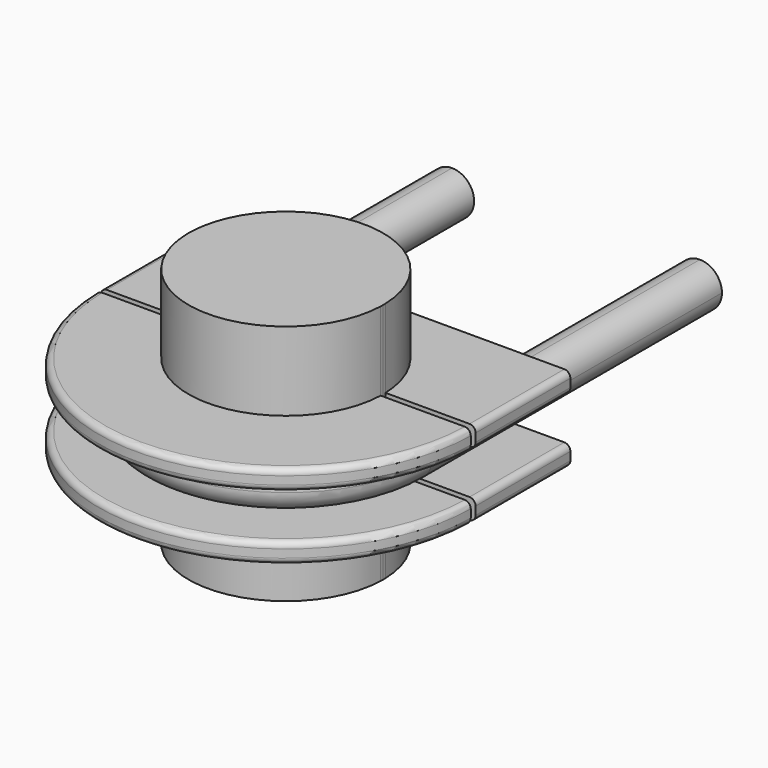
from build123d import *

# Parameters (mm, degrees)
F0_W          = 10.4959674797
F0_H          = 19.6
F4_DEPTH      = 7
F4_DEPTH_BACK = 7
F6_R          = 1
F6_2_R        = 1


with BuildPart() as f2:
    # F2: sweep along a path in F0
    with BuildLine(Plane.XY) as f2_path:
        Line((-20.5, 60), (-20.5, 0))
        ThreePointArc((-20.5, 0), (0, -20.5), (20.5, 0))
        Line((20.5, 0), (20.5, 60))
    # F1 (on Front) → F2 (sweep)
    with BuildSketch(Plane.XZ):
        with BuildLine():
            ThreePointArc((20.5, -3.65), (23.0809397513, -2.5809397513), (24.15, 0))
            ThreePointArc((24.15, 0), (23.0809397513, 2.5809397513), (20.5, 3.65))
            ThreePointArc((20.5, 3.65), (16.85, 0), (20.5, -3.65))
        make_face()
    sweep(path=f2_path.line)


with BuildPart() as f3:
    # F3: sweep along a path in F1
    with BuildLine(Plane.XZ) as f3_path:
        Line((0, -20), (0, 0))
        Line((0, 0), (0, 20))
    # F0 (on Top) → F3 (sweep)
    with BuildSketch(Plane.XY):
        with BuildLine():
            ThreePointArc((-16.0922341519, 0.5), (-16.1, 0), (-16.0922341519, -0.5))
            Line((-16.0922341519, -0.5), (16.0922341519, -0.5))
            ThreePointArc((16.0922341519, -0.5), (16.0980584209, -0.2500301524), (16.1, 0))
            ThreePointArc((16.1, 0), (16.0980584209, 0.2500301524), (16.0922341519, 0.5))
            Line((16.0922341519, 0.5), (-16.0922341519, 0.5))
        make_face()
        with BuildLine():
            ThreePointArc((16.0922341519, 0.5), (0, 16.1), (-16.0922341519, 0.5))
            Line((-16.0922341519, 0.5), (16.0922341519, 0.5))
        make_face()
        with BuildLine():
            Line((16.0922341519, -0.5), (-16.0922341519, -0.5))
            ThreePointArc((-16.0922341519, -0.5), (0, -16.1), (16.0922341519, -0.5))
        make_face()
    sweep(path=f3_path.line)


with BuildPart() as f4:
    # F0 (on Top) → F4 (new body, two sides)
    with BuildSketch(Plane.XY) as f4_sk:
        with BuildLine():
            Line((-20.5, 20.1), (-20.5, 0.5))
            Line((-20.5, 0.5), (-16.0922341519, 0.5))
            ThreePointArc((-16.0922341519, 0.5), (0, 16.1), (16.0922341519, 0.5))
            Line((16.0922341519, 0.5), (20.5, 0.5))
            Line((20.5, 0.5), (20.5, 20.1))
            Line((20.5, 20.1), (-20.5, 20.1))
        make_face()
        with Locations((-25.7479837398, 10.3)):
            Rectangle(F0_W, F0_H)
        with Locations((25.7479837398, 10.3)):
            Rectangle(F0_W, F0_H)
    extrude(amount=F4_DEPTH)
    extrude(f4_sk.sketch, amount=-F4_DEPTH_BACK)


with BuildPart() as f4b:
    # F0 (on Top) → F4, piece 2 (new body, two sides)
    with BuildSketch(Plane.XY) as f4_2_sk:
        with BuildLine():
            Line((-16.0922341519, -0.5), (-20.4939015319, -0.5))
            ThreePointArc((-20.4939015319, -0.5), (0, -20.5), (20.4939015319, -0.5))
            Line((20.4939015319, -0.5), (16.0922341519, -0.5))
            ThreePointArc((16.0922341519, -0.5), (0, -16.1), (-16.0922341519, -0.5))
        make_face()
        with BuildLine():
            ThreePointArc((20.4939015319, -0.5), (0, -20.5), (-20.4939015319, -0.5))
            Line((-20.4939015319, -0.5), (-30.9959674797, -0.5))
            ThreePointArc((-30.9959674797, -0.5), (0, -31), (30.9959674797, -0.5))
            Line((30.9959674797, -0.5), (20.4939015319, -0.5))
        make_face()
    extrude(amount=F4_DEPTH)
    extrude(f4_2_sk.sketch, amount=-F4_DEPTH_BACK)


with BuildPart() as f5_tool:
    # F5: sweep along a path in F0
    with BuildLine(Plane.XY) as f5_path:
        Line((20.5, 60), (20.5, 0))
        ThreePointArc((20.5, 0), (0, -20.5), (-20.5, 0))
        Line((-20.5, 0), (-20.5, 60))
    # F1 (on Front) → F5 (sweep)
    with BuildSketch(Plane.XZ):
        with BuildLine():
            ThreePointArc((20.5, -3.65), (23.0809397513, -2.5809397513), (24.15, 0))
            ThreePointArc((24.15, 0), (23.0809397513, 2.5809397513), (20.5, 3.65))
            ThreePointArc((20.5, 3.65), (16.85, 0), (20.5, -3.65))
        make_face()
        with BuildLine():
            ThreePointArc((20.5, 3.65), (23.0809397513, 2.5809397513), (24.15, 0))
            ThreePointArc((24.15, 0), (23.0809397513, -2.5809397513), (20.5, -3.65))
            Line((20.5, -3.65), (31.2, -3.65))
            Line((31.2, -3.65), (31.2, 3.65))
            Line((31.2, 3.65), (20.5, 3.65))
        make_face()
    sweep(path=f5_path.line)


with BuildPart() as f4_1:
    add(f4.part)

    # F5: cut by f5_tool
    add(f5_tool.part, mode=Mode.SUBTRACT)

    # F6
    f6_edges = [f4_1.edges().sort_by_distance(p)[0] for p in [
        (30.995967, 10.3, 7),
        (30.995967, 10.3, 3.65),
        (30.995967, 10.3, -7),
        (-30.995967, 10.3, 7),
        (-30.995967, 10.3, -7),
        (-30.995967, 10.3, 3.65),
        (-30.995967, 10.3, -3.65),
        (30.995967, 10.3, -3.65),
    ]]
    fillet(f6_edges, radius=F6_R)


with BuildPart() as f4b_1:
    add(f4b.part)

    # F5: cut by f5_tool
    add(f5_tool.part, mode=Mode.SUBTRACT)

    # F6#2
    f6_2_edges = [f4b_1.edges().sort_by_distance(p)[0] for p in [
        (0, -31, -7),
        (0, -31, 7),
        (0, -31, -3.65),
        (0, -31, 3.65),
    ]]
    fillet(f6_2_edges, radius=F6_2_R)


solid = Compound([f2.part, f3.part, f4_1.part, f4b_1.part])
